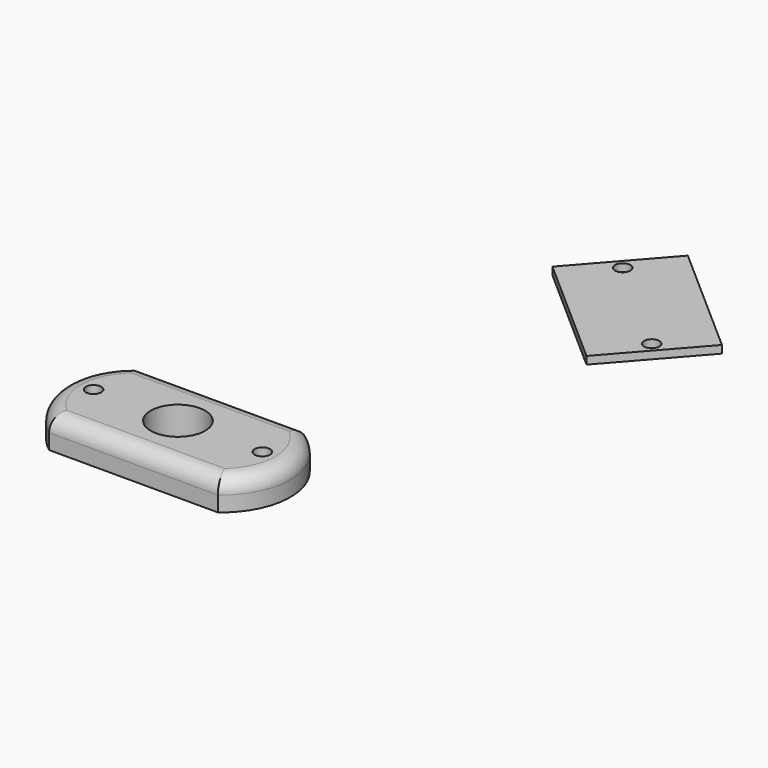
from build123d import *

# Parameters (mm, degrees)
F0_R        = 1
F1_DEPTH    = 1
F2_W        = 22
F2_H        = 14.5
F3_DEPTH    = 4
F4_R        = 1
F4_R_2      = 3.55
F5_DEPTH    = 5
F6_T1_DEPTH = 32
F6_T4_ANGLE = 171.0262354859
F6_T6_ANGLE = 171.0262354859


# Not quite as in the source:
# - a fillet or chamfer that OpenCascade refuses, or shapes differently, is made with other operations: its cross-section is extruded or revolved along the edge and cut away or added


with BuildPart() as f1:
    # F0 (on Top) → F1 (new body)
    with BuildSketch(Plane.XY):
        Polygon((-15.7937894361, 8.8500456174), (-30.8080597745, 22.0626035153), (-40.056850303, 11.5526142783), (-25.0425799646, -1.6599436195), align=None)
        with Locations((-21.5442549757, 4.5859928413)):
            Circle(F0_R, mode=Mode.SUBTRACT)
        with Locations((-34.3063847634, 15.8166670545)):
            Circle(F0_R, mode=Mode.SUBTRACT)
    extrude(amount=F1_DEPTH)


with BuildPart() as f3:
    # F2 (on Top) → F3 (new body)
    with BuildSketch(Plane.XY):
        with Locations((-45, -43.2913755476)):
            Rectangle(F2_W, F2_H)
        with BuildLine():
            ThreePointArc((-34, -50.5413755476), (-30.3326822519, -43.2913755476), (-34, -36.0413755476))
            Line((-34, -36.0413755476), (-34, -50.5413755476))
        make_face()
        with BuildLine():
            Line((-56, -50.5413755476), (-56, -36.0413755476))
            ThreePointArc((-56, -36.0413755476), (-59.6673177481, -43.2913755476), (-56, -50.5413755476))
        make_face()
    extrude(amount=F3_DEPTH)

    # F4 (on face) → F5 (cut)
    with BuildSketch(Plane.XY.offset(4)):
        with Locations((-56, -43.2913755476)):
            Circle(F4_R)
        with Locations((-34, -43.2913755476)):
            Circle(F4_R)
        with Locations((-45, -43.2913755476)):
            Circle(F4_R_2)
    extrude(amount=-F5_DEPTH, mode=Mode.SUBTRACT)

    # F6: fillet of radius 2 on 4 edges, made by hand

    # F6_s2 → F6_t1 (cut)
    with BuildSketch(Plane.YZ.offset(-61)):
        with BuildLine():
            ThreePointArc((-48.5413755476, 4), (-49.95558911, 3.4142135624), (-50.5413755476, 2))
            Line((-50.5413755476, 2), (-50.5413755476, 4))
            Line((-50.5413755476, 4), (-48.5413755476, 4))
        make_face()
        with BuildLine():
            ThreePointArc((-36.0413755476, 2), (-36.6271619853, 3.4142135624), (-38.0413755476, 4))
            Line((-38.0413755476, 4), (-36.0413755476, 4))
            Line((-36.0413755476, 4), (-36.0413755476, 2))
        make_face()
    extrude(amount=F6_T1_DEPTH, mode=Mode.SUBTRACT)

    # F6_s3 → F6_t4 (revolve, cut)
    with BuildSketch(Plane(origin=(-53.7335722058, -4.2165456866, 0), x_dir=(0, 0, 1), z_dir=(0.9969352706, 0.0782308516, 0))):
        with BuildLine():
            ThreePointArc((2, 30.1949517804), (3.4142135624, 30.7807382181), (4, 32.1949517804))
            Line((4, 32.1949517804), (4, 30.1949517804))
            Line((4, 30.1949517804), (2, 30.1949517804))
        make_face()
    revolve(axis=Axis((-50.6673177481, -43.2913755476, 4), (0, 0, 1)), revolution_arc=F6_T4_ANGLE, mode=Mode.SUBTRACT)

    # F6_s5 → F6_t6 (revolve, cut)
    with BuildSketch(Plane(origin=(-42.4683054286, -3.33254505, 0), x_dir=(0, 0, 1), z_dir=(-0.9969352706, -0.0782308516, 0))):
        with BuildLine():
            ThreePointArc((2, -49.0816699683), (3.4142135624, -48.4958835307), (4, -47.0816699683))
            Line((4, -47.0816699683), (4, -49.0816699683))
            Line((4, -49.0816699683), (2, -49.0816699683))
        make_face()
    revolve(axis=Axis((-39.3326822519, -43.2913755476, 4), (0, 0, 1)), revolution_arc=F6_T6_ANGLE, mode=Mode.SUBTRACT)


solid = Compound([f1.part, f3.part])
